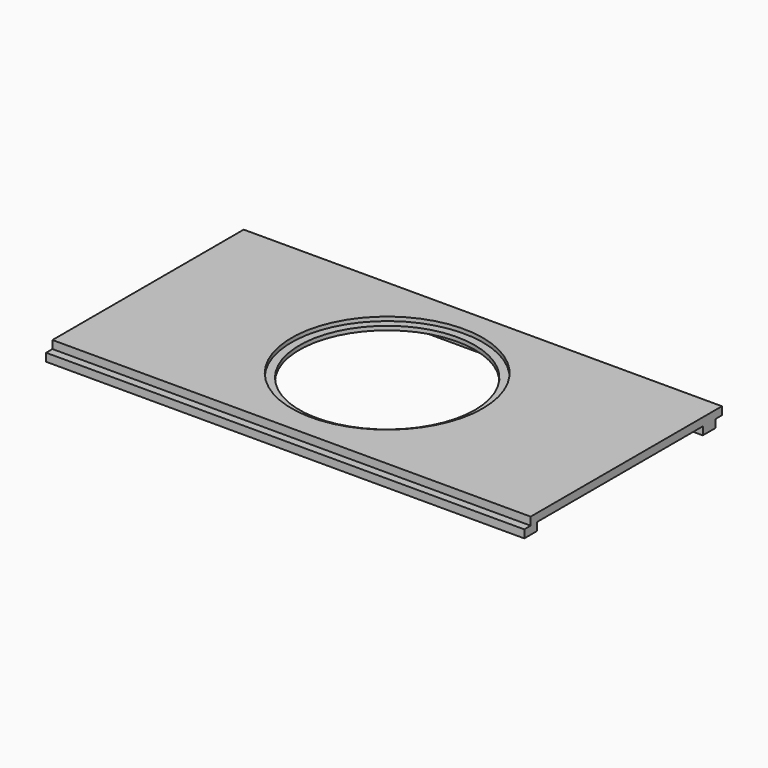
from build123d import *

# Parameters (mm, degrees)
F0_W     = 600
F0_H     = 300
F0_R     = 120
F1_DEPTH = 10
F0_R_2   = 110
F2_DEPTH = 5
F3_W     = 600
F3_H     = 10
F4_DEPTH = 10


# Not quite as in the source:
# - a feature names something its author has since deleted; it is built from what else it names


with BuildPart() as f1:
    # F0 (on Top) → F1 (new body)
    with BuildSketch(Plane.XY):
        Rectangle(F0_W, F0_H)
        Circle(F0_R, mode=Mode.SUBTRACT)
    extrude(amount=F1_DEPTH)

    # F0 (on Top) → F2 (join)
    with BuildSketch(Plane.XY):
        Circle(F0_R)
        Circle(F0_R_2, mode=Mode.SUBTRACT)
    extrude(amount=F2_DEPTH)

    # F3 (on face) → F4 (join)
    with BuildSketch(Plane.XY):
        with Locations((0, -145)):
            Rectangle(F3_W, F3_H)
        with Locations((0, -155)):
            Rectangle(F3_W, F3_H)
        Polygon((300, 140), (-300, 140), (-300, 120), (-9.09e-08, 120), (300, 120), align=None)
    extrude(amount=-F4_DEPTH)


solid = f1.part
